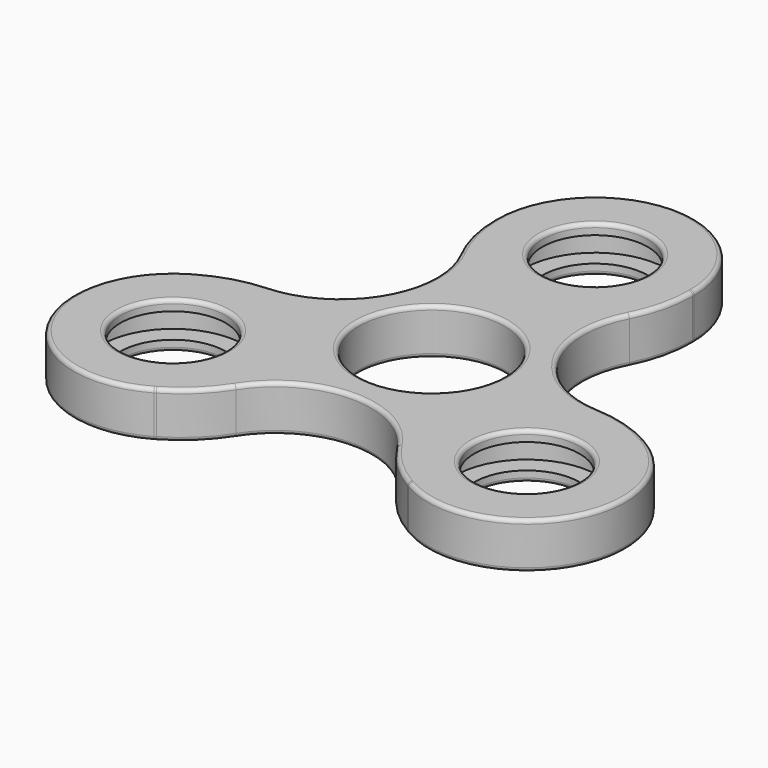
from build123d import *

# Parameters (mm, degrees)
F0_R             = 15.05
F0_R_2           = 11.05
F1_DEPTH         = 7
F2_R             = 10.8
F3_DEPTH         = 7
F3_COPIES_COUNT  = 3
F5_DEPTH         = 118
F5_COPIES_COUNT  = 3
F6_R             = 20
F7_R             = 10.8
F7_R_2           = 8
F8_DEPTH         = 1.6
F8_COPIES_COUNT  = 3
F9_R             = 10.8
F9_R_2           = 8
F10_DEPTH        = 1.6
F10_COPIES_COUNT = 3
F11_R            = 0.6


# Not quite as in the source:
# - two fillets or chamfers of one size are made in one step
# - an extrude ends at something that could not be found from the text; its depth is read off the source's solid
# - a pattern or mirror of a feature is missing from the dataset's text; its kind, count and spacing are read off the source's solid


with BuildPart() as f1:
    # F0 (on Top) → F1 (new body)
    with BuildSketch(Plane.XY):
        Circle(F0_R)
        Circle(F0_R_2, mode=Mode.SUBTRACT)
    extrude(amount=F1_DEPTH)

    # F2 (on Top) → F3 (join, through all)
    with BuildSketch(Plane.XY):
        with BuildLine():
            Line((15.05, 0), (15.05, 31))
            ThreePointArc((15.05, 31), (0, 46.05), (-15.05, 31))
            Line((-15.05, 31), (-15.05, 0))
            ThreePointArc((-15.05, 0), (0, 15.05), (15.05, 0))
        make_face()
        with Locations((0, 31)):
            Circle(F2_R, mode=Mode.SUBTRACT)
    f3 = extrude(amount=F3_DEPTH)

    # F3_copies: F3 ×3 about axis
    f3_copies_axis = Axis((0, 0, 0), (0, 0, 1))
    for i in range(1, F3_COPIES_COUNT):
        add(f3.rotate(f3_copies_axis, i * 360 / F3_COPIES_COUNT))

    # F4 (on Top) → F5 (cut, through all)
    with BuildSketch(Plane.XY):
        with BuildLine():
            Line((15.05, 8.6891215513), (15.05, 24.6891215513))
            ThreePointArc((15.05, 24.6891215513), (13.1204970221, 7.5751224876), (28.9064064606, 0.6891215513))
            Line((28.9064064606, 0.6891215513), (15.05, 8.6891215513))
        make_face()
    f5 = extrude(amount=F5_DEPTH, mode=Mode.SUBTRACT)

    # F5_copies: F5 ×3 about axis
    f5_copies_axis = Axis((0, 0, 0), (0, 0, 1))
    for i in range(1, F5_COPIES_COUNT):
        add(f5.rotate(f5_copies_axis, i * 360 / F5_COPIES_COUNT), mode=Mode.SUBTRACT)

    # F6
    f6_edges = [f1.edges().sort_by_distance(p)[0] for p in [
        (15.05, 24.689122, 3.5),
        (28.906406, 0.689122, 3.5),
        (13.856406, -25.378243, 3.5),
        (-13.856406, -25.378243, 3.5),
        (-28.906406, 0.689122, 3.5),
        (-15.05, 24.689122, 3.5),
    ]]
    fillet(f6_edges, radius=F6_R)

    # F7 (on Top) → F8 (join)
    with BuildSketch(Plane.XY):
        with Locations((26.8467875173, -15.5)):
            Circle(F7_R)
        with Locations((26.8467875173, -15.5)):
            Circle(F7_R_2, mode=Mode.SUBTRACT)
    f8 = extrude(amount=F8_DEPTH)

    # F8_copies: F8 ×3 about axis
    f8_copies_axis = Axis((0, 0, 0), (0, 0, 1))
    for i in range(1, F8_COPIES_COUNT):
        add(f8.rotate(f8_copies_axis, i * 360 / F8_COPIES_COUNT))

    # F9 (on face) → F10 (join)
    with BuildSketch(Plane.XY.offset(7)):
        with Locations((26.8467875173, -15.5)):
            Circle(F9_R)
        with Locations((26.8467875173, -15.5)):
            Circle(F9_R_2, mode=Mode.SUBTRACT)
    f10 = extrude(amount=-F10_DEPTH)

    # F10_copies: F10 ×3 about axis
    f10_copies_axis = Axis((0, 0, 0), (0, 0, 1))
    for i in range(1, F10_COPIES_COUNT):
        add(f10.rotate(f10_copies_axis, i * 360 / F10_COPIES_COUNT))

    # F11
    f11_edges = [f1.edges().sort_by_distance(p)[0] for p in [
        (-11.05, 0, 7),
        (-11.05, 0, 0),
        (34.244231, -2.392673, 7),
        (29.728941, -0.443118, 7),
        (13.120497, 7.575122, 7),
        (14.480719, 25.967577, 7),
        (15.05, 30.85271, 7),
        (0, 46.05, 7),
        (-15.05, 30.85271, 7),
        (-14.480719, 25.967577, 7),
        (-13.120497, 7.575122, 7),
        (-29.728941, -0.443118, 7),
        (-34.244231, -2.392673, 7),
        (-39.88047, -23.025, 7),
        (-19.194231, -28.460037, 7),
        (-15.248222, -25.524459, 7),
        (0, -15.150245, 7),
        (15.248222, -25.524459, 7),
        (19.194231, -28.460037, 7),
        (39.88047, -23.025, 7),
        (18.846788, -15.5, 7),
        (4, 24.071797, 7),
        (-22.846788, -8.571797, 7),
        (-22.846788, -8.571797, 0),
        (13.120497, 7.575122, 0),
        (14.480719, 25.967577, 0),
        (15.05, 30.85271, 0),
        (0, 46.05, 0),
        (-15.05, 30.85271, 0),
        (-14.480719, 25.967577, 0),
        (-13.120497, 7.575122, 0),
        (-29.728941, -0.443118, 0),
        (-34.244231, -2.392673, 0),
        (-39.88047, -23.025, 0),
        (-19.194231, -28.460037, 0),
        (-15.248222, -25.524459, 0),
        (0, -15.150245, 0),
        (15.248222, -25.524459, 0),
        (19.194231, -28.460037, 0),
        (39.88047, -23.025, 0),
        (34.244231, -2.392673, 0),
        (29.728941, -0.443118, 0),
        (18.846788, -15.5, 0),
        (4, 24.071797, 0),
    ]]
    fillet(f11_edges, radius=F11_R)


solid = f1.part
